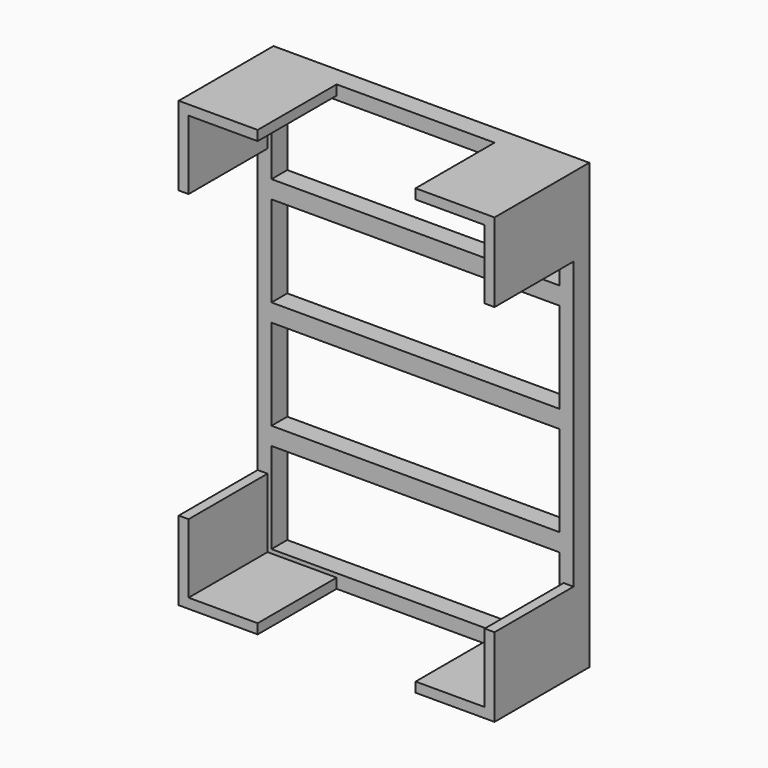
from build123d import *

# Parameters (mm, degrees)
F0_W     = 203.2
F0_H     = 285.75
F0_W_2   = 190.5
F0_H_2   = 63.5
F0_W_3   = 185.42
F0_H_3   = 58.42
F1_DEPTH = 12.7
F3_W     = 6.35
F3_H     = 6.35
F3_W_2   = 44.45
F3_H_2   = 44.45
F4_DEPTH = 63.5


# Not quite as in the source:
# - the program builds the solid bodies; features that only make, move or delete a surface that nothing else refers to are left out


with BuildPart() as f1:
    # F0 (on Front) → F1 (new body)
    with BuildSketch(Plane.XZ):
        Rectangle(F0_W, F0_H)
        with Locations((0, -104.775)):
            Rectangle(F0_W_2, F0_H_2, mode=Mode.SUBTRACT)
        with Locations((0, -34.925)):
            Rectangle(F0_W_2, F0_H_2, mode=Mode.SUBTRACT)
        with Locations((0, 34.925)):
            Rectangle(F0_W_2, F0_H_2, mode=Mode.SUBTRACT)
        with Locations((0, 104.775)):
            Rectangle(F0_W_2, F0_H_2, mode=Mode.SUBTRACT)
        with Locations((0, 104.775)):
            Rectangle(F0_W_2, F0_H_2)
        with Locations((0, 104.775)):
            Rectangle(F0_W_3, F0_H_3, mode=Mode.SUBTRACT)
        with Locations((0, 34.925)):
            Rectangle(F0_W_2, F0_H_2)
        with Locations((0, 34.925)):
            Rectangle(F0_W_3, F0_H_3, mode=Mode.SUBTRACT)
        with Locations((0, -34.925)):
            Rectangle(F0_W_2, F0_H_2)
        with Locations((0, -34.925)):
            Rectangle(F0_W_3, F0_H_3, mode=Mode.SUBTRACT)
        with Locations((0, -104.775)):
            Rectangle(F0_W_2, F0_H_2)
        with Locations((0, -104.775)):
            Rectangle(F0_W_3, F0_H_3, mode=Mode.SUBTRACT)
    extrude(amount=F1_DEPTH)

    # F3 (on face) → F4 (join)
    with BuildSketch(Plane.XZ.offset(12.7)):
        with Locations((98.425, -139.7)):
            Rectangle(F3_W, F3_H)
        with Locations((73.025, -139.7)):
            Rectangle(F3_W_2, F3_H)
        with Locations((98.425, -114.3)):
            Rectangle(F3_W, F3_H_2)
        with Locations((98.425, 114.3)):
            Rectangle(F3_W, F3_H_2)
        with Locations((98.425, 139.7)):
            Rectangle(F3_W, F3_H)
        with Locations((73.025, 139.7)):
            Rectangle(F3_W_2, F3_H)
        with Locations((-98.425, -139.7)):
            Rectangle(F3_W, F3_H)
        with Locations((-73.025, -139.7)):
            Rectangle(F3_W_2, F3_H)
        with Locations((-98.425, -114.3)):
            Rectangle(F3_W, F3_H_2)
        with Locations((-98.425, 114.3)):
            Rectangle(F3_W, F3_H_2)
        with Locations((-98.425, 139.7)):
            Rectangle(F3_W, F3_H)
        with Locations((-73.025, 139.7)):
            Rectangle(F3_W_2, F3_H)
    extrude(amount=F4_DEPTH)


solid = f1.part
